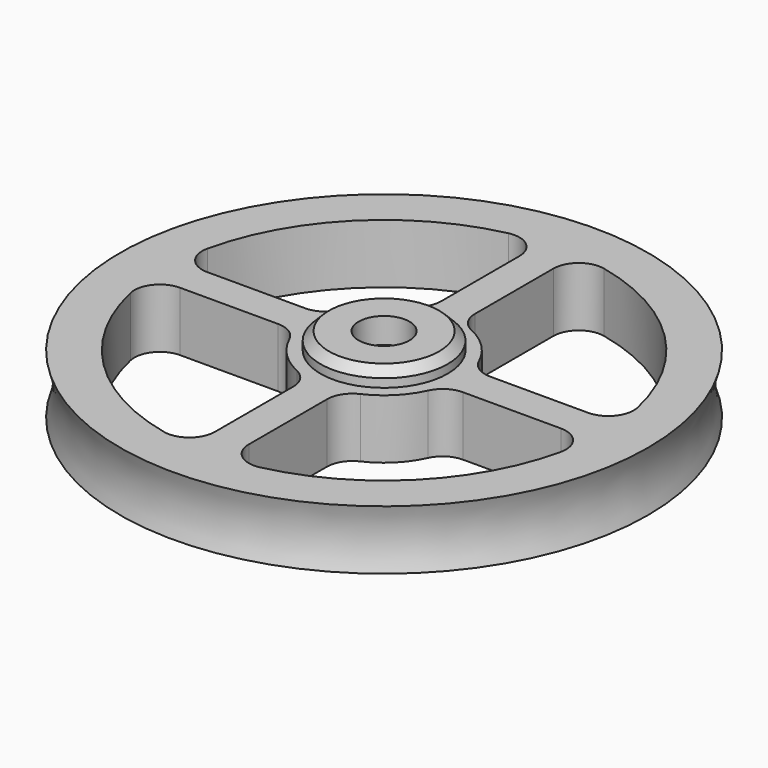
from build123d import *

# Parameters (mm, degrees)
F0_R             = 30
F0_R_2           = 1.5
F1_DEPTH         = 2
F2_R             = 7.5
F2_R_2           = 1.5
F3_DEPTH         = 2
F4_R             = 3
F4_R_2           = 1.5
F5_DEPTH         = 3
F6_SIZE          = 1
F7_R             = 30
F7_R_2           = 4
F8_DEPTH         = 5
F10_DEPTH        = 25
F10_COPIES_COUNT = 4
F11_R            = 3


# Not quite as in the source:
# - a pattern or mirror of a feature is missing from the dataset's text; its kind, count and spacing are read off the source's solid


with BuildPart() as f1:
    # F0 (on Top) → F1 (new body)
    with BuildSketch(Plane.XY):
        Circle(F0_R)
        Circle(F0_R_2, mode=Mode.SUBTRACT)
    extrude(amount=F1_DEPTH)

    # F2 (on face) → F3 (join)
    with BuildSketch(Plane.XY.offset(2)):
        Circle(F2_R)
        Circle(F2_R_2, mode=Mode.SUBTRACT)
    extrude(amount=F3_DEPTH)

    # F4 (on face) → F5 (cut)
    with BuildSketch(Plane.XY.offset(4)):
        Circle(F4_R)
        Circle(F4_R_2, mode=Mode.SUBTRACT)
    extrude(amount=-F5_DEPTH, mode=Mode.SUBTRACT)

    # F6
    f6_edges = [f1.edges().sort_by_distance(p)[0] for p in [
        (-7.5, 0, 4),
    ]]
    chamfer(f6_edges, length=F6_SIZE)

    # F7 (on face) → F8 (join)
    with BuildSketch(Plane(origin=(0, 0, 0), x_dir=(1, 0, 0), z_dir=(0, 0, -1))):
        Circle(F7_R)
        Circle(F7_R_2, mode=Mode.SUBTRACT)
    extrude(amount=F8_DEPTH)

    # F9 (on face) → F10 (cut)
    with BuildSketch(Plane.XY.offset(2)):
        with BuildLine():
            Line((2, -8.7749643874), (2, -25.9229627936))
            ThreePointArc((2, -25.9229627936), (18.3847763109, -18.3847763109), (25.9229627936, -2))
            Line((25.9229627936, -2), (8.7749643874, -2))
            ThreePointArc((8.7749643874, -2), (6.3639610307, -6.3639610307), (2, -8.7749643874))
        make_face()
    f10 = extrude(amount=-F10_DEPTH, mode=Mode.SUBTRACT)

    # F10_copies: F10 ×4 about axis
    f10_copies_axis = Axis((0, 0, 0), (0, 0, 1))
    for i in range(1, F10_COPIES_COUNT):
        add(f10.rotate(f10_copies_axis, i * 360 / F10_COPIES_COUNT), mode=Mode.SUBTRACT)

    # F11
    f11_edges = [f1.edges().sort_by_distance(p)[0] for p in [
        (8.774964, -2, -1.5),
        (2, -25.922963, -1.5),
        (25.922963, -2, -1.5),
        (2, -8.774964, -1.5),
        (-2, -8.774964, -1.5),
        (-2, -25.922963, -1.5),
        (-8.774964, -2, -1.5),
        (-25.922963, -2, -1.5),
        (-8.774964, 2, -1.5),
        (-25.922963, 2, -1.5),
        (-2, 25.922963, -1.5),
        (-2, 8.774964, -1.5),
        (2, 8.774964, -1.5),
        (2, 25.922963, -1.5),
        (25.922963, 2, -1.5),
        (8.774964, 2, -1.5),
    ]]
    fillet(f11_edges, radius=F11_R)

    # F12 (on Front) → F13 (revolve)
    with BuildSketch(Plane.XZ):
        with BuildLine():
            Line((31.1325030024, 2), (30, 2))
            Line((30, 2), (30, -5))
            Line((30, -5), (31.1325030024, -5))
            ThreePointArc((31.1325030024, -5), (30.5, -1.5), (31.1325030024, 2))
        make_face()
    revolve(axis=Axis((0, 0, 4), (0, 0, 1)))


solid = f1.part
